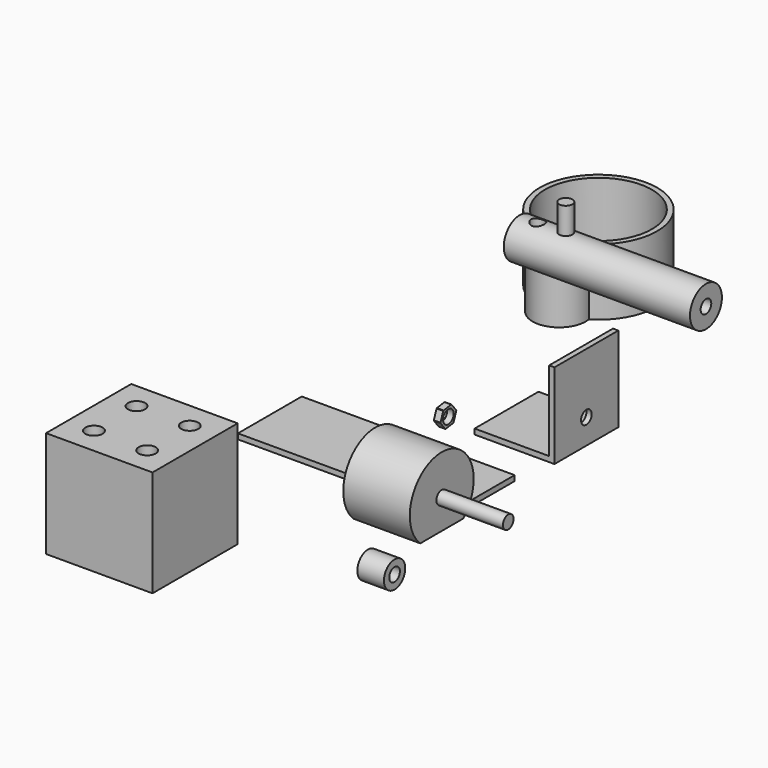
from build123d import *

# Parameters (mm, degrees)
F0_W      = 30
F0_H      = 30
F1_DEPTH  = 2
F2_W      = 2
F2_H      = 30
F3_DEPTH  = 30
F5_DEPTH  = 25
F6_R      = 2.5
F7_DEPTH  = 25
F8_R      = 2.5
F9_DEPTH  = 2
F0_W_2    = 80
F10_DEPTH = 2
F12_DEPTH = 2.5
F4_R      = 5
F4_R_2    = 2.5
F13_DEPTH = 10
F14_DEPTH = 25
F0_W_3    = 40
F0_H_2    = 40
F15_DEPTH = 40
F16_R     = 3.2254140047
F17_DEPTH = 5
F18_R     = 2.5
F19_DEPTH = 70
F22_DEPTH = 91.6849308292
F23_DEPTH = 10


# Not quite as in the source:
# - a feature names something its author has since deleted; it is built from what else it names


with BuildPart() as f1:
    # F0 (on Top) → F1 (new body)
    with BuildSketch(Plane.XY):
        with Locations((5.4872950528, 30.7764774188)):
            Rectangle(F0_W, F0_H)
    extrude(amount=F1_DEPTH)

    # F2 (on face) → F3 (join)
    with BuildSketch(Plane.XY.offset(2)):
        with Locations((19.4872950528, 30.7764774188)):
            Rectangle(F2_W, F2_H)
    extrude(amount=F3_DEPTH)

    # F8 (on face) → F9 (cut, through all)
    with BuildSketch(Plane(origin=(18.4872950528, 0, 0), x_dir=(0, -1, 0), z_dir=(-1, 0, 0))):
        with Locations((-30.7764774188, 9.41)):
            Circle(F8_R)
    extrude(amount=-F9_DEPTH, mode=Mode.SUBTRACT)


with BuildPart() as f5:
    # F4 (on Right) → F5 (new body)
    with BuildSketch(Plane.YZ):
        with BuildLine():
            Line((-52.8934156308, 3.1420226926), (-32.7376361042, 3.1420226926))
            ThreePointArc((-32.7376361042, 3.1420226926), (-42.8155258675, 29.2522044156), (-52.8934156308, 3.1420226926))
        make_face()
    extrude(amount=F5_DEPTH)

    # F6 (on face) → F7 (join)
    with BuildSketch(Plane.YZ.offset(25)):
        with Locations((-42.8155258675, 14.2522044156)):
            Circle(F6_R)
    extrude(amount=F7_DEPTH)


with BuildPart() as f10:
    # F0 (on Top) → F10 (new body)
    with BuildSketch(Plane.XY):
        with Locations((-21.8575587869, -15)):
            Rectangle(F0_W_2, F0_H)
    extrude(amount=F10_DEPTH)


with BuildPart() as f12:
    # F6 (on face) → F12 (new body)
    with BuildSketch(Plane.YZ.offset(25)):
        with BuildLine():
            Line((-39.1193990775, 42.3947411596), (-41.3449491195, 45.2110034407))
            ThreePointArc((-41.3449491195, 45.2110034407), (-41.4300421528, 45.2460511048), (-41.5159695959, 45.27900012))
            Line((-41.5159695959, 45.27900012), (-45.0676992959, 44.7597483868))
            ThreePointArc((-45.0676992959, 44.7597483868), (-45.1405979801, 44.7035794904), (-45.2120963858, 44.6456386494))
            Line((-45.2120963858, 44.6456386494), (-46.538276044, 41.3101246351))
            ThreePointArc((-46.538276044, 41.3101246351), (-46.5260816948, 41.2189080745), (-46.5116526575, 41.1280182183))
            Line((-46.5116526575, 41.1280182183), (-44.2861026155, 38.3117559373))
            ThreePointArc((-44.2861026155, 38.3117559373), (-44.2010095822, 38.2767082732), (-44.1150821391, 38.2437592579))
            Line((-44.1150821391, 38.2437592579), (-40.563352439, 38.7630109911))
            ThreePointArc((-40.563352439, 38.7630109911), (-40.4904537549, 38.8191798876), (-40.4189553491, 38.8771207286))
            Line((-40.4189553491, 38.8771207286), (-39.092775691, 42.2126347428))
            ThreePointArc((-39.092775691, 42.2126347428), (-39.1049700402, 42.3038513034), (-39.1193990775, 42.3947411596))
        make_face()
        with Locations((-42.8155258675, 41.761379689)):
            Circle(F6_R, mode=Mode.SUBTRACT)
    extrude(amount=F12_DEPTH)


with BuildPart() as f13:
    # F4 (on Right) → F13 (new body)
    with BuildSketch(Plane.YZ):
        with Locations((-46.217340976, -14.7316996008)):
            Circle(F4_R)
        with Locations((-46.217340976, -14.7316996008)):
            Circle(F4_R_2, mode=Mode.SUBTRACT)
    extrude(amount=F13_DEPTH)


with BuildPart() as f14:
    # F0 (on Top) → F14 (new body)
    with BuildSketch(Plane.XY):
        with BuildLine():
            ThreePointArc((-29.0589361801, 93.8513494414), (-42.2885690725, 134.7708941054), (-48.9334039126, 92.2823251494))
            ThreePointArc((-48.9334039126, 92.2823251494), (-38.1463908298, 82.3028805443), (-29.0589361801, 93.8513494414))
        make_face()
        with BuildLine():
            ThreePointArc((-46.8168556195, 93.6324783746), (-42.1311653612, 132.7770977087), (-31.361124685, 94.8526578336))
            ThreePointArc((-31.361124685, 94.8526578336), (-38.303794541, 84.2966769411), (-46.8168556195, 93.6324783746))
        make_face(mode=Mode.SUBTRACT)
    extrude(amount=F14_DEPTH)


with BuildPart() as f15:
    # F0 (on Top) → F15 (new body)
    with BuildSketch(Plane.XY):
        with Locations((-40.3018663824, -102.0636367798)):
            Rectangle(F0_W_3, F0_H_2)
    extrude(amount=F15_DEPTH)

    # F16 (on face) → F17 (cut)
    with BuildSketch(Plane.XY.offset(40)):
        with Locations((-50.3018663824, -112.0636367798)):
            Circle(F16_R)
        with Locations((-30.3018663824, -112.0636367798)):
            Circle(F16_R)
        with Locations((-30.3018663824, -92.0636367798)):
            Circle(F16_R)
        with Locations((-50.3018663824, -92.0636367798)):
            Circle(F16_R)
    extrude(amount=-F17_DEPTH, mode=Mode.SUBTRACT)


with BuildPart() as f19:
    # F18 (on Right) → F19 (new body)
    with BuildSketch(Plane.YZ):
        with BuildLine():
            ThreePointArc((25.0680372119, 71.9522312284), (19.764736353, 59.1489303695), (32.5680372119, 64.4522312284))
            ThreePointArc((32.5680372119, 64.4522312284), (30.3713380708, 69.7555320873), (25.0680372119, 71.9522312284))
        make_face()
        with Locations((25.0680372119, 64.4522312284)):
            Circle(F18_R, mode=Mode.SUBTRACT)
    extrude(amount=F19_DEPTH)

    # F21 (on face) → F22 (cut, through all)
    with BuildSketch(Plane(origin=(0, 0, 71.9522312284), x_dir=(1, 0, 0), z_dir=(0, 0, -1))):
        with BuildLine():
            Line((4.2916242406, -25.0680372119), (9.2916242406, -25.0680372119))
            ThreePointArc((9.2916242406, -25.0680372119), (6.7916242406, -22.5680372119), (4.2916242406, -25.0680372119))
        make_face()
        with BuildLine():
            ThreePointArc((4.2916242406, -25.0680372119), (6.7916242406, -27.5680372119), (9.2916242406, -25.0680372119))
            Line((9.2916242406, -25.0680372119), (4.2916242406, -25.0680372119))
        make_face()
    extrude(amount=F22_DEPTH, mode=Mode.SUBTRACT)


with BuildPart() as f23:
    # F21 (on face) → F23 (new body)
    with BuildSketch(Plane(origin=(0, 0, 71.9522312284), x_dir=(1, 0, 0), z_dir=(0, 0, -1))):
        with BuildLine():
            ThreePointArc((19.8193216324, -25.0680372119), (17.3193216324, -22.5680372119), (14.8193216324, -25.0680372119))
            Line((14.8193216324, -25.0680372119), (19.8193216324, -25.0680372119))
        make_face()
        with BuildLine():
            Line((19.8193216324, -25.0680372119), (14.8193216324, -25.0680372119))
            ThreePointArc((14.8193216324, -25.0680372119), (17.3193216324, -27.5680372119), (19.8193216324, -25.0680372119))
        make_face()
    extrude(amount=-F23_DEPTH)


solid = Compound([f1.part, f5.part, f10.part, f12.part, f13.part, f14.part, f15.part, f19.part, f23.part])
